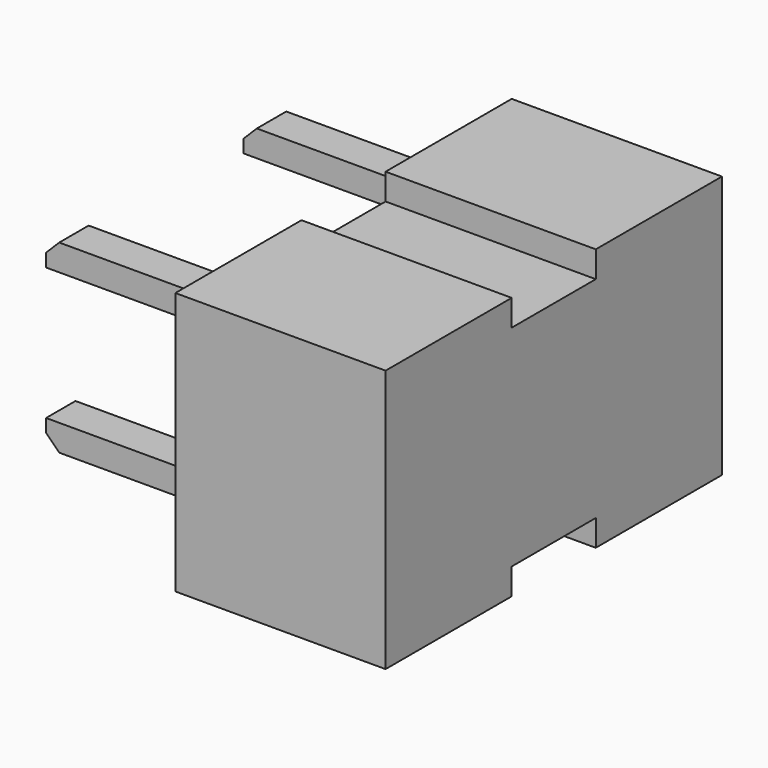
from build123d import *

# Parameters (mm, degrees)
F1_DEPTH = 50.8
F3_DEPTH = 8.89


with BuildPart() as f1:
    # F0 (on Right) → F1 (new body)
    with BuildSketch(Plane.YZ):
        Polygon((12.7, 25.4), (0, 25.4), (-12.7, 25.4), (-12.7, 31.75), (-50.8, 31.75), (-50.8, 0), (-50.8, -31.75), (-12.7, -31.75), (-12.7, -25.4), (0, -25.4), (12.7, -25.4), (12.7, -31.75), (50.8, -31.75), (50.8, 0), (50.8, 31.75), (12.7, 31.75), align=None)
    extrude(amount=F1_DEPTH)


with BuildPart() as f3:
    # F2 (on Front) → F3 (new body)
    with BuildSketch(Plane.XZ):
        Polygon((0, 19.05), (0, 25.4), (-41.275, 25.4), (-44.45, 22.225), (-44.45, 19.05), align=None)
    extrude(amount=F3_DEPTH)


with BuildPart() as f4_1:
    # F4: instance of F3
    add(f3.part.mirror(Plane.XY))


with BuildPart() as f3_1:
    # F5: moved
    add(f3.part.moved(Location((0, -38.1, 0))))


with BuildPart() as f4_1_1:
    # F5: moved
    add(f4_1.part.moved(Location((0, -38.1, 0))))


with BuildPart() as f3_2:
    # F6: moved
    add(f3_1.part.moved(Location((0, 0, 5.08))))


with BuildPart() as f4_1_2:
    # F7: moved
    add(f4_1_1.part.moved(Location((0, 0, -5.08))))


with BuildPart() as f8_1:
    # F8: instance of F3
    add(f3_2.part.mirror(Plane.XZ))


with BuildPart() as f8_2:
    # F8: instance of F4_1
    add(f4_1_2.part.mirror(Plane.XZ))


with BuildPart() as f3_3:
    # F9: moved
    add(f3_2.part.moved(Location((0, 0, -8.128))))


with BuildPart() as f8_1_1:
    # F10: moved
    add(f8_1.part.moved(Location((0, 0, -8.128))))


with BuildPart() as f8_2_1:
    # F11: moved
    add(f8_2.part.moved(Location((0, 0, 8.128))))


with BuildPart() as f4_1_3:
    # F11: moved
    add(f4_1_2.part.moved(Location((0, 0, 8.128))))


with BuildPart() as f3_4:
    # F12: moved
    add(f3_3.part.moved(Location((0, 12.7, 0))))


with BuildPart() as f4_1_4:
    # F12: moved
    add(f4_1_3.part.moved(Location((0, 12.7, 0))))


with BuildPart() as f8_1_2:
    # F13: moved
    add(f8_1_1.part.moved(Location((0, -12.7, 0))))


with BuildPart() as f8_2_2:
    # F13: moved
    add(f8_2_1.part.moved(Location((0, -12.7, 0))))


solid = Compound([f1.part, f3_4.part, f4_1_4.part, f8_1_2.part, f8_2_2.part])
